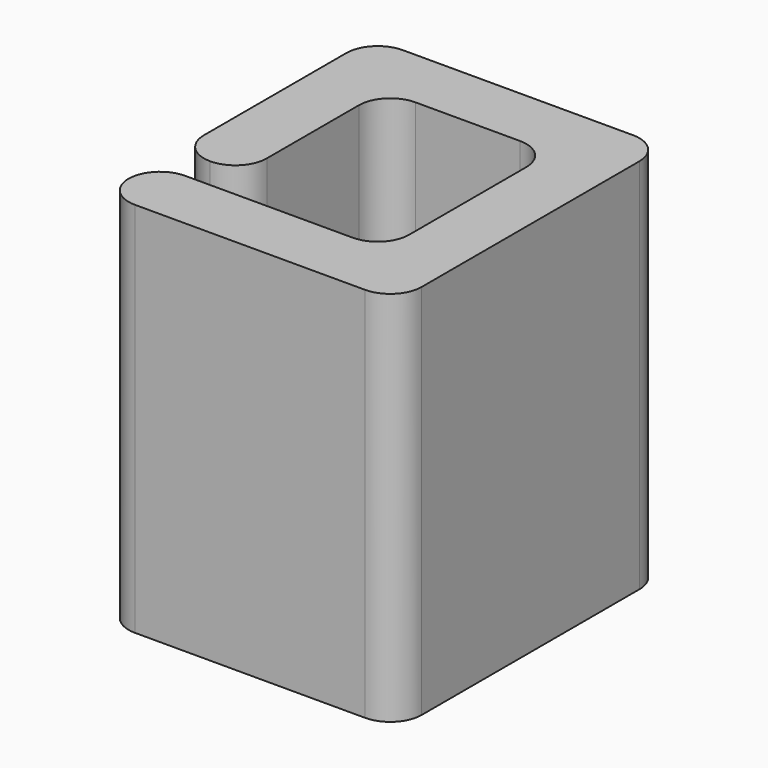
from build123d import *

# Parameters (mm, degrees)
F0_W     = 14
F0_H     = 18
F1_DEPTH = 3
F2_W     = 3
F2_H     = 8.5
F2_H_2   = 10
F3_DEPTH = 18
F4_R     = 1.49999


# Not quite as in the source:
# - a fillet or chamfer is up to 0.001 mm smaller than in the source, because OpenCascade refuses the exact size


with BuildPart() as f1:
    # F0 (on Front) → F1 (new body)
    with BuildSketch(Plane.XZ):
        with Locations((7, 9)):
            Rectangle(F0_W, F0_H)
    extrude(amount=F1_DEPTH)

    # F2 (on face) → F3 (join, through all)
    with BuildSketch(Plane.XY.offset(18)):
        with Locations((1.5, -7.25)):
            Rectangle(F2_W, F2_H)
        Polygon((3, -13), (0, -13), (0, -16), (14, -16), (14, -13), (11, -13), align=None)
        with Locations((12.5, -8)):
            Rectangle(F2_W, F2_H_2)
    extrude(amount=-F3_DEPTH)

    # F4 (radius 1.5 in the source; OpenCascade refuses exactly that, so slightly less here)
    f4_edges = [f1.edges().sort_by_distance(p)[0] for p in [
        (0, -11.5, 9),
        (0, -13, 9),
        (0, -16, 9),
        (3, -11.5, 9),
        (14, -16, 9),
        (14, 0, 9),
        (0, 0, 9),
        (3, -3, 9),
        (11, -3, 9),
        (11, -13, 9),
    ]]
    fillet(f4_edges, radius=F4_R)


solid = f1.part
